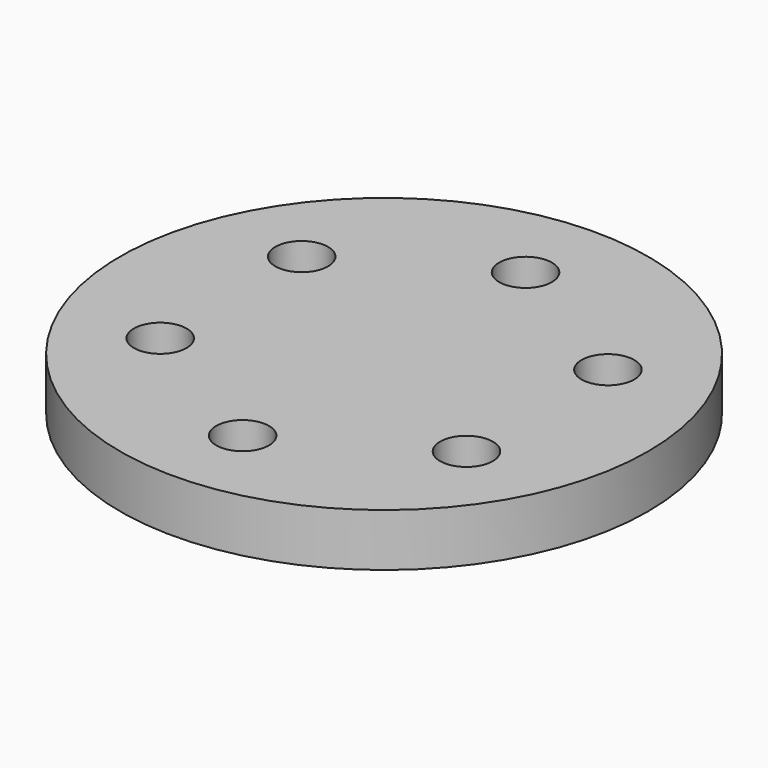
from build123d import *

# Parameters (mm, degrees)
F2_R            = 60
F3_DEPTH        = 12
F5_R            = 6
F6_DEPTH        = 12.001
F6_COPIES_COUNT = 6


# Not quite as in the source:
# - a pattern or mirror of a feature is missing from the dataset's text; its kind, count and spacing are read off the source's solid


with BuildPart() as f3:
    # F2 (on Top) → F3 (new body)
    with BuildSketch(Plane.XY):
        Circle(F2_R)
    extrude(amount=F3_DEPTH)

    # F5 (on face) → F6 (cut, through all)
    with BuildSketch(Plane.XY.offset(12)):
        with Locations((0, 40.1915311813)):
            Circle(F5_R)
    f6 = extrude(amount=-F6_DEPTH, mode=Mode.SUBTRACT)

    # F6_copies: F6 ×6 about axis
    f6_copies_axis = Axis((0, 0, 0), (0, 0, 1))
    for i in range(1, F6_COPIES_COUNT):
        add(f6.rotate(f6_copies_axis, i * 360 / F6_COPIES_COUNT), mode=Mode.SUBTRACT)


solid = f3.part
